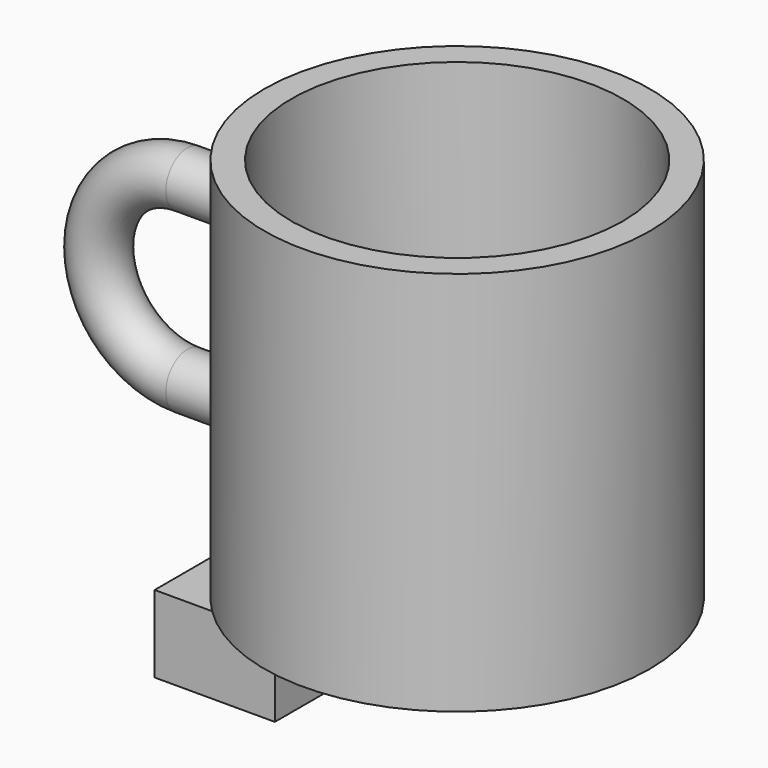
from build123d import *

# Parameters (mm, degrees)
F0_R     = 63.5
F1_DEPTH = 127
F2_R     = 54.61
F3_DEPTH = 114.3
F4_W     = 39.6098716408
F4_H     = 45.2183522284
F5_DEPTH = 25.4
F6_R     = 8.89
F7_DEPTH = 25.4
F8_R     = 8.89
F9_ANGLE = 180


with BuildPart() as f1:
    # F0 (on Top) → F1 (new body)
    with BuildSketch(Plane.XY):
        Circle(F0_R)
    extrude(amount=F1_DEPTH)

    # F2 (on face) → F3 (cut)
    with BuildSketch(Plane.XY.offset(127)):
        Circle(F2_R)
    extrude(amount=-F3_DEPTH, mode=Mode.SUBTRACT)

    # F4 (on face) → F5 (join)
    with BuildSketch(Plane(origin=(0, 0, 0), x_dir=(1, 0, 0), z_dir=(0, 0, -1))):
        with Locations((-43.6950641796, 22.6091761142)):
            Rectangle(F4_W, F4_H)
    extrude(amount=F5_DEPTH)


with BuildPart() as f7:
    # F6 (on face) → F7 (new body)
    with BuildSketch(Plane(origin=(-63.5, 0, 0), x_dir=(0, -1, 0), z_dir=(-1, 0, 0))):
        with Locations((0, 92.71)):
            Circle(F6_R)
    extrude(amount=F7_DEPTH)

    # F8 (on face) → F9 (revolve)
    with BuildSketch(Plane(origin=(-88.9, 0, 0), x_dir=(0, -1, 0), z_dir=(-1, 0, 0))):
        with Locations((0, 92.71)):
            Circle(F8_R)
    revolve(axis=Axis((-88.9, 0.4127491266, 63.5), (0, -1, 0)), revolution_arc=F9_ANGLE)


with BuildPart() as f7b:
    # F6 (on face) → F7, piece 2 (new body)
    with BuildSketch(Plane(origin=(-63.5, 0, 0), x_dir=(0, -1, 0), z_dir=(-1, 0, 0))):
        with Locations((0, 34.29)):
            Circle(F6_R)
    extrude(amount=F7_DEPTH)


solid = Compound([f1.part, f7.part, f7b.part])
